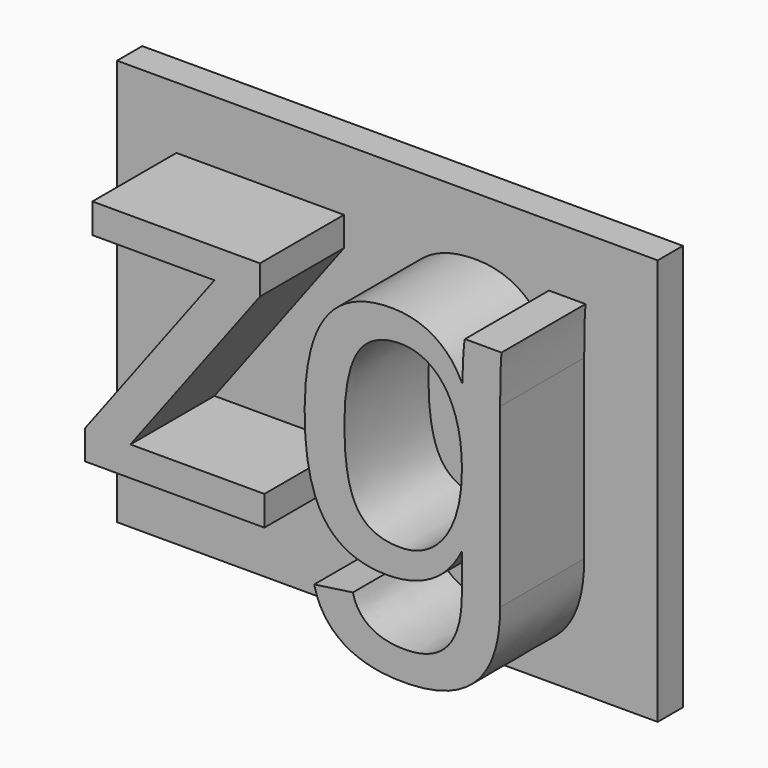
from build123d import *

# Parameters (mm, degrees)
F0_TEXT_SIZE = 105.8333333333
F1_DEPTH     = 25.4
F2_W         = 130.7261809707
F2_H         = 98.2439089566
F3_DEPTH     = 7.62


# Not quite as in the source:
# - Text() gives the source's letters only with a copy of the font that has no kerning and outlines rounded to 1/6400 em; it was checked with that copy


with BuildPart() as f1:
    # F0 (on Front) → F1 (new body)
    with BuildSketch(Plane.XZ):
        with Locations((-50.6793365001, -43.9824225939)):
            Text('zg', F0_TEXT_SIZE, font='Arimo', text_align=(TextAlign.LEFT, TextAlign.BOTTOM))
    extrude(amount=F1_DEPTH)

    # F2 (on Front) → F3 (join)
    with BuildSketch(Plane.XZ):
        with Locations((6.376888603, -22.2194632515)):
            Rectangle(F2_W, F2_H)
    extrude(amount=-F3_DEPTH)


solid = f1.part
